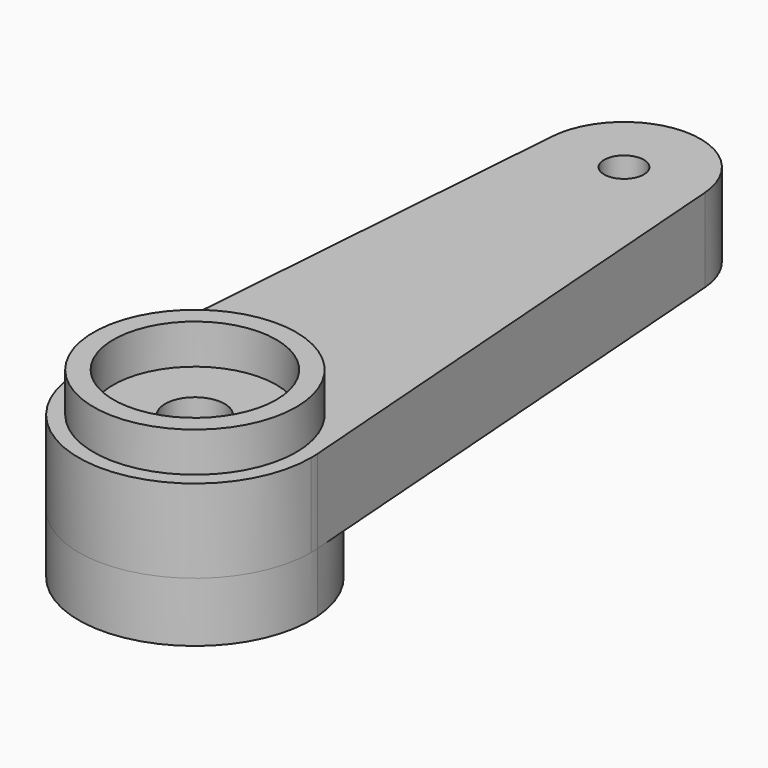
from build123d import *
from build123d import SkipClean  # not in build123d's __all__

# Parameters (mm, degrees)
F0_R     = 0.75
F0_R_2   = 0.5
F1_DEPTH = 2.1
F2_R     = 1.85
F3_DEPTH = 1.5
F4_R     = 2.55
F4_R_2   = 2.05
F5_DEPTH = 1


# Not quite as in the source:
# - after a boolean that leaves OpenCascade's solid faulty, fix() repairs it


with BuildPart() as f1:
    # F0 (on Top) → F1 (new body)
    with BuildSketch(Plane.XY):
        with BuildLine():
            ThreePointArc((-2.9169642705, 0.2166666667), (-0.108407815, -2.9229903773), (2.925, 0))
            ThreePointArc((2.925, 0), (2.9229903773, 0.108407815), (2.9169642705, 0.2166666667))
            ThreePointArc((2.9169642705, 0.2166666667), (0, 2.925), (-2.9169642705, 0.2166666667))
        make_face()
        Circle(F0_R, mode=Mode.SUBTRACT)
        with BuildLine():
            ThreePointArc((-2.9169642705, 0.2166666667), (0, 2.925), (2.9169642705, 0.2166666667))
            Line((2.9169642705, 0.2166666667), (1.9197115285, 13.6425925926))
            ThreePointArc((1.9197115285, 13.6425925926), (1.9236774278, 13.5713453141), (1.925, 13.5))
            ThreePointArc((1.925, 13.5), (-0.0713453141, 11.5763225722), (-1.9197115285, 13.6425925926))
            Line((-1.9197115285, 13.6425925926), (-2.9169642705, 0.2166666667))
        make_face()
        with BuildLine():
            ThreePointArc((1.925, 13.5), (1.9236774278, 13.5713453141), (1.9197115285, 13.6425925926))
            ThreePointArc((1.9197115285, 13.6425925926), (0, 15.425), (-1.9197115285, 13.6425925926))
            ThreePointArc((-1.9197115285, 13.6425925926), (-0.0713453141, 11.5763225722), (1.925, 13.5))
        make_face()
        with Locations((0, 13.5)):
            Circle(F0_R_2, mode=Mode.SUBTRACT)
    extrude(amount=F1_DEPTH)

    # F2 (on face) → F3 (join)
    with BuildSketch(Plane.XY):
        with BuildLine():
            ThreePointArc((2.9169642705, 0.2166666667), (0, 2.925), (-2.9169642705, 0.2166666667))
            ThreePointArc((-2.9169642705, 0.2166666667), (0, -2.925), (2.9169642705, 0.2166666667))
        make_face()
        Circle(F2_R, mode=Mode.SUBTRACT)
    with SkipClean():  # cleaning this boolean's faces spoils the solid; the shape is the same uncleaned
        extrude(amount=-F3_DEPTH)

    # F4 (on face) → F5 (join)
    with BuildSketch(Plane.XY.offset(2.1)):
        Circle(F4_R)
        Circle(F4_R_2, mode=Mode.SUBTRACT)
    extrude(amount=F5_DEPTH)

    add(f1.part.fix(), mode=Mode.REPLACE)


solid = f1.part
